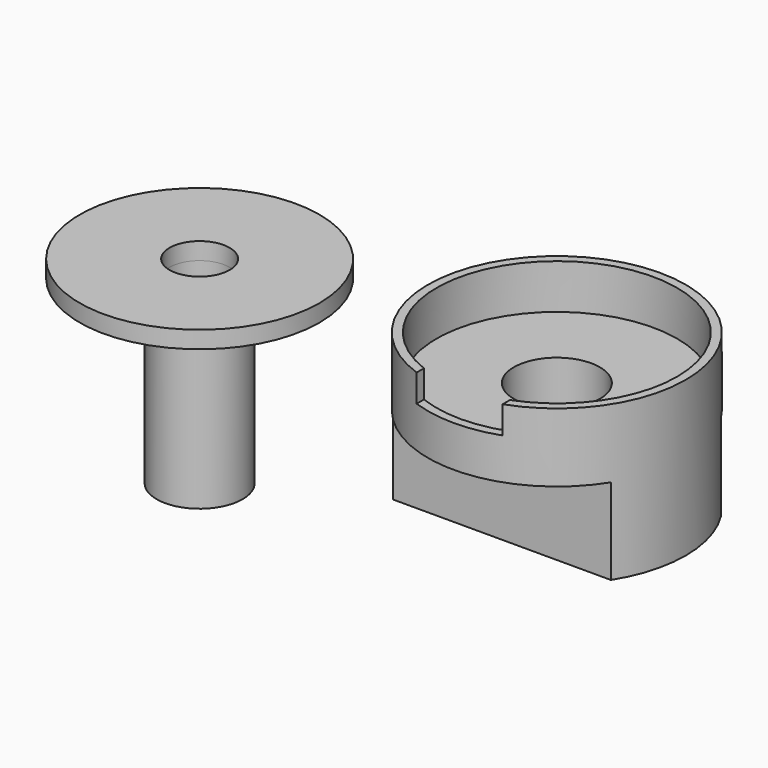
from build123d import *

# Parameters (mm, degrees)
F0_R     = 6.975
F0_R_2   = 2.5
F0_R_3   = 1.75
F1_DEPTH = 1
F2_DEPTH = 10.5
F5_W     = 5
F5_H     = 1.6
F6_DEPTH = 7.501
F8_DEPTH = 5


# Not quite as in the source:
# - a feature names something its author has since deleted; it is built from what else it names


with BuildPart() as f1:
    # F0 (on Top) → F1 (new body)
    with BuildSketch(Plane.XY):
        Circle(F0_R)
        Circle(F0_R_2, mode=Mode.SUBTRACT)
        Circle(F0_R_2)
        Circle(F0_R_3, mode=Mode.SUBTRACT)
    extrude(amount=F1_DEPTH)

    # F0 (on Top) → F2 (join)
    with BuildSketch(Plane.XY):
        Circle(F0_R_2)
        Circle(F0_R_3, mode=Mode.SUBTRACT)
    extrude(amount=-F2_DEPTH)


with BuildPart() as f4:
    # F3 (on Front) → F4 (revolve)
    with BuildSketch(Plane.XZ):
        Polygon((28.2853133976, -5), (28.2853133976, 4), (27.7853133976, 4), (27.7853133976, 1.4), (23.2853133976, 1.4), (23.2853133976, -5), align=None)
    revolve(axis=Axis((20.7853133976, 0, -0.6741590851), (0, 0, -1)))

    # F5 (on Front) → F6 (cut, through all)
    with BuildSketch(Plane.XZ):
        with Locations((20.7853133976, 3.2)):
            Rectangle(F5_W, F5_H)
    extrude(amount=F6_DEPTH, mode=Mode.SUBTRACT)

    # F7 (on face) → F8 (cut)
    with BuildSketch(Plane(origin=(0, 0, -5), x_dir=(1, 0, 0), z_dir=(0, 0, -1))):
        with BuildLine():
            ThreePointArc((27.1296021679, 4), (20.7853133976, 7.5), (14.4410246274, 4))
            Line((14.4410246274, 4), (27.1296021679, 4))
        make_face()
        with BuildLine():
            Line((27.1296021679, -4), (14.4410246274, -4))
            ThreePointArc((14.4410246274, -4), (20.7853133976, -7.5), (27.1296021679, -4))
        make_face()
    extrude(amount=-F8_DEPTH, mode=Mode.SUBTRACT)


solid = Compound([f1.part, f4.part])
